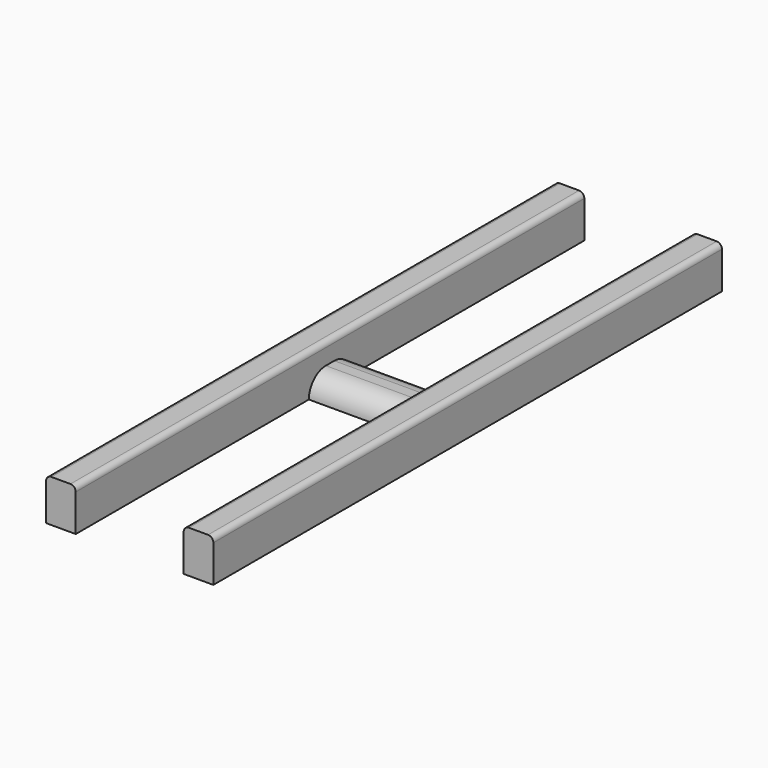
from build123d import *

# Parameters (mm, degrees)
F1_DEPTH = 76.2
F0_W     = 25.8755748077
F0_H     = 5.08
F2_DEPTH = 6.35
F3_R     = 1.27
F4_R     = 5.07999


# Not quite as in the source:
# - two fillets or chamfers of one size are made in one step
# - a fillet or chamfer is up to 0.001 mm smaller than in the source, because OpenCascade refuses the exact size


with BuildPart() as f1:
    # F0 (on Front) → F1 (new body, symmetric)
    with BuildSketch(Plane.XZ):
        Polygon((-38.5863832052, 10.16), (-45.6983832052, 10.16), (-45.6983832052, 0), (-38.5863832052, 0), (-38.5863832052, 5.08), align=None)
    extrude(amount=F1_DEPTH, both=True)



with BuildPart() as f1b:
    # F0 (on Front) → F1, piece 2 (new body, symmetric)
    with BuildSketch(Plane.XZ):
        Polygon((-12.7108083974, 10.16), (-12.7108083974, 5.08), (-12.7108083974, 0), (-5.5988083974, 0), (-5.5988083974, 10.16), align=None)
    extrude(amount=F1_DEPTH, both=True)


with BuildPart() as f1_1:
    add(f1.part)

    add(f1b.part)  # F2 merges F1b
    # F0 (on Front) → F2 (join, symmetric)
    with BuildSketch(Plane.XZ):
        Polygon((-38.5863832052, 10.16), (-45.6983832052, 10.16), (-45.6983832052, 0), (-38.5863832052, 0), (-38.5863832052, 5.08), align=None)
        with Locations((-25.6485958013, 2.54)):
            Rectangle(F0_W, F0_H)
        Polygon((-12.7108083974, 10.16), (-12.7108083974, 5.08), (-12.7108083974, 0), (-5.5988083974, 0), (-5.5988083974, 10.16), align=None)
    extrude(amount=F2_DEPTH, both=True)

    # F3
    f3_edges = [f1_1.edges().sort_by_distance(p)[0] for p in [
        (-45.698383, 0, 10.16),
        (-38.586383, 0, 10.16),
        (-12.710808, 0, 10.16),
        (-5.598808, 0, 10.16),
    ]]
    fillet(f3_edges, radius=F3_R)

    # F4 (radius 5.08 in the source; OpenCascade refuses exactly that, so slightly less here)
    f4_edges = [f1_1.edges().sort_by_distance(p)[0] for p in [
        (-25.648596, 6.35, 5.08),
        (-25.648596, -6.35, 5.08),
    ]]
    fillet(f4_edges, radius=F4_R)


solid = f1_1.part
